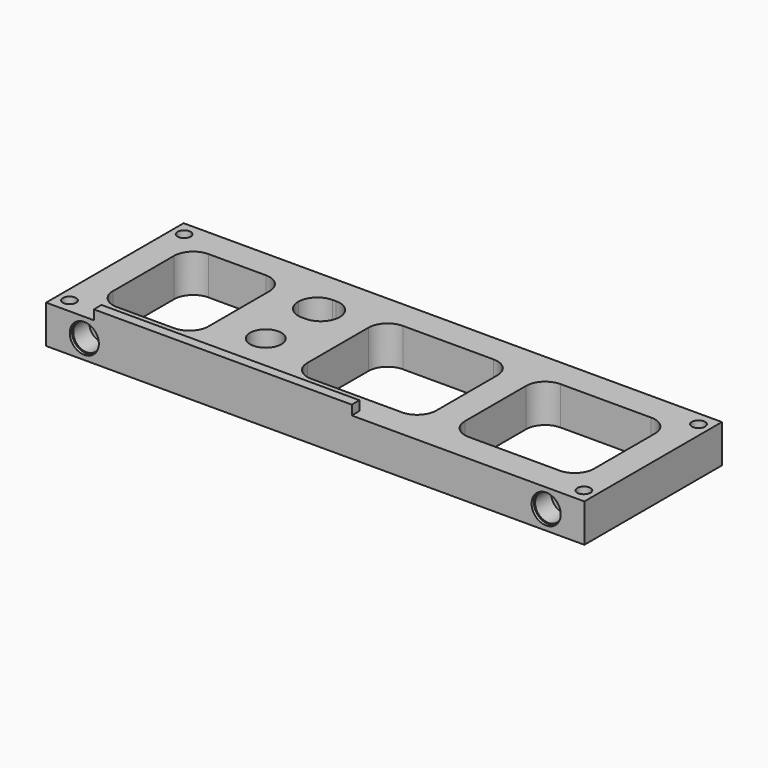
from build123d import *

# Parameters (mm, degrees)
F0_W      = 112.7
F0_H      = 36
F1_DEPTH  = 8
F3_W      = 54
F3_H      = 2
F4_DEPTH  = 2
F5_R      = 3.27
F6_DEPTH  = 8.001
F7_R      = 1.375
F8_DEPTH  = 10.001
F10_R     = 5.25
F11_DEPTH = 4.5
F9_W      = 20
F9_H      = 24
F9_W_2    = 27
F9_W_3    = 8.7
F9_H_2    = 8
F12_DEPTH = 10.001
F13_R     = 3.99999
F14_R     = 2.795
F15_DEPTH = 4.8
F16_R     = 2.795
F17_DEPTH = 4.8
F18_R     = 3.05
F19_DEPTH = 0.6
F20_R     = 3.05
F21_DEPTH = 0.6


# Not quite as in the source:
# - a fillet or chamfer is up to 0.001 mm smaller than in the source, because OpenCascade refuses the exact size


with BuildPart() as f1:
    # F0 (on Top) → F1 (new body)
    with BuildSketch(Plane.XY):
        Rectangle(F0_W, F0_H)
    extrude(amount=F1_DEPTH)

    # F3 (on face) → F4 (join)
    with BuildSketch(Plane.XY.offset(8)):
        with Locations((-19.35, -17)):
            Rectangle(F3_W, F3_H)
    extrude(amount=F4_DEPTH)

    # F5 (on face) → F6 (cut, through all)
    with BuildSketch(Plane.XY.offset(8)):
        with Locations((-20.35, -5.5)):
            Circle(F5_R)
    extrude(amount=-F6_DEPTH, mode=Mode.SUBTRACT)

    # F7 (on face) → F8 (cut, through all)
    with BuildSketch(Plane(origin=(0, 0, 0), x_dir=(1, 0, 0), z_dir=(0, 0, -1))):
        with Locations((-53.85, 15)):
            Circle(F7_R)
        with Locations((-53.85, -15)):
            Circle(F7_R)
        with Locations((53.85, 15)):
            Circle(F7_R)
        with Locations((53.85, -15)):
            Circle(F7_R)
    extrude(amount=-F8_DEPTH, mode=Mode.SUBTRACT)

    # F10 (on face) → F11 (cut)
    with BuildSketch(Plane(origin=(0, 0, 0), x_dir=(1, 0, 0), z_dir=(0, 0, -1))):
        with Locations((-20.35, 5.5)):
            Circle(F10_R)
    extrude(amount=-F11_DEPTH, mode=Mode.SUBTRACT)

    # F9 (on face) → F12 (cut, through all)
    with BuildSketch(Plane(origin=(0, 0, 0), x_dir=(1, 0, 0), z_dir=(0, 0, -1))):
        with Locations((-40.35, 0)):
            Rectangle(F9_W, F9_H)
        with Locations((3.85, 0)):
            Rectangle(F9_W_2, F9_H)
        with Locations((36.85, 0)):
            Rectangle(F9_W_2, F9_H)
        with Locations((-20, -8)):
            Rectangle(F9_W_3, F9_H_2)
    extrude(amount=-F12_DEPTH, mode=Mode.SUBTRACT)

    # F13 (radius 4 in the source; OpenCascade refuses exactly that, so slightly less here)
    f13_edges = [f1.edges().sort_by_distance(p)[0] for p in [
        (-30.35, -12, 4),
        (-50.35, -12, 4),
        (-50.35, 12, 4),
        (-30.35, 12, 4),
        (-24.35, 4, 4),
        (-9.65, -12, 4),
        (23.35, -12, 4),
        (-9.65, 12, 4),
        (-24.35, 12, 4),
        (17.35, -12, 4),
        (50.35, -12, 4),
        (50.35, 12, 4),
        (23.35, 12, 4),
        (-15.65, 4, 4),
        (-15.65, 12, 4),
        (17.35, 12, 4),
    ]]
    fillet(f13_edges, radius=F13_R)

    # F14 (on face) → F15 (cut)
    with BuildSketch(Plane.XZ.offset(18)):
        with Locations((48.35, 4)):
            Circle(F14_R)
        with Locations((-48.35, 4)):
            Circle(F14_R)
    extrude(amount=-F15_DEPTH, mode=Mode.SUBTRACT)

    # F16 (on face) → F17 (cut)
    with BuildSketch(Plane(origin=(0, 18, 0), x_dir=(-1, 0, 0), z_dir=(0, 1, 0))):
        with Locations((48.35, 4)):
            Circle(F16_R)
        with Locations((-48.35, 4)):
            Circle(F16_R)
    extrude(amount=-F17_DEPTH, mode=Mode.SUBTRACT)

    # F18 (on face) → F19 (cut)
    with BuildSketch(Plane.XZ.offset(18)):
        with Locations((-48.35, 4)):
            Circle(F18_R)
        with Locations((48.35, 4)):
            Circle(F18_R)
    extrude(amount=-F19_DEPTH, mode=Mode.SUBTRACT)

    # F20 (on face) → F21 (cut)
    with BuildSketch(Plane(origin=(0, 18, 0), x_dir=(-1, 0, 0), z_dir=(0, 1, 0))):
        with Locations((-48.35, 4)):
            Circle(F20_R)
        with Locations((48.35, 4)):
            Circle(F20_R)
    extrude(amount=-F21_DEPTH, mode=Mode.SUBTRACT)


solid = f1.part
